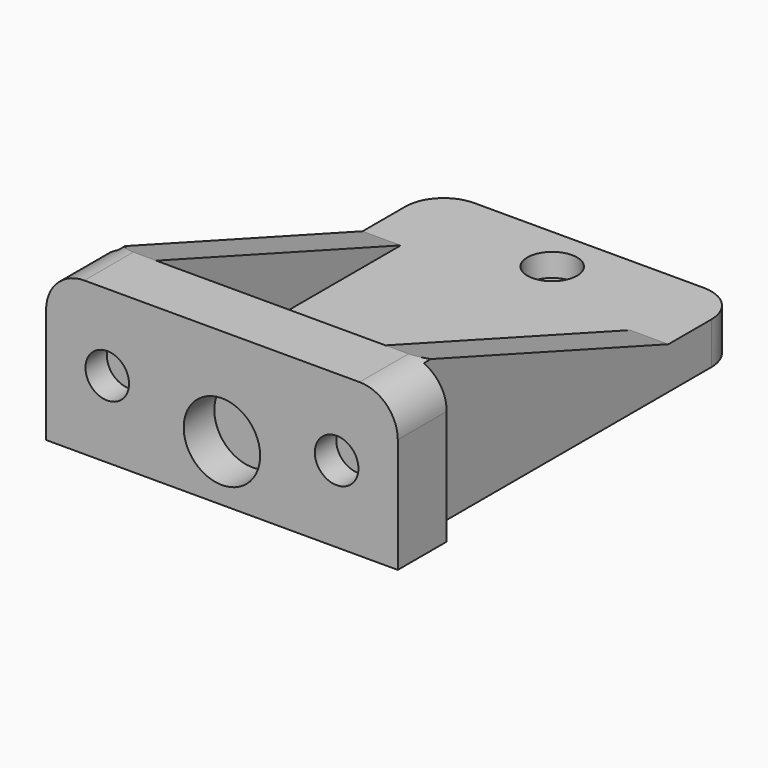
from build123d import *

# Parameters (mm, degrees)
F0_W           = 3
F0_H           = 8
F1_DEPTH       = 20
F0_W_2         = 30
F0_H_2         = 12
F0_H_3         = 40
F0_W_3         = 5
F2_DEPTH       = 5.5
F3_DEPTH       = 20
F5_DEPTH       = 43.001
F7_D           = 3.3
F7_DEPTH       = 13.5002857143
F7_CBORE_D     = 6.5
F7_CBORE_DEPTH = 3
F7_TIP         = 0.9914200214
F8_R           = 5
F9_DEPTH       = 5
F8_R_2         = 2.85
F10_DEPTH      = 3.5
F11_T1_DEPTH   = 30.5
F11_T3_DEPTH   = 33


# Not quite as in the source:
# - a fillet or chamfer that OpenCascade refuses, or shapes differently, is made with other operations: its cross-section is extruded or revolved along the edge and cut away or added


with BuildPart() as f1:
    # F0 (on Top) → F1 (new body)
    with BuildSketch(Plane.XY):
        Polygon((20, -30), (20, -22), (15, -22), (-15, -22), (-20, -22), (-20, -30), align=None)
        with Locations((-21.5, -26)):
            Rectangle(F0_W, F0_H)
        with Locations((21.5, -26)):
            Rectangle(F0_W, F0_H)
    extrude(amount=F1_DEPTH)

    # F0 (on Top) → F2 (join)
    with BuildSketch(Plane.XY):
        with Locations((0, 24)):
            Rectangle(F0_W_2, F0_H_2)
        with Locations((0, -2)):
            Rectangle(F0_W_2, F0_H_3)
        with Locations((-17.5, 24)):
            Rectangle(F0_W_3, F0_H_2)
        with Locations((-17.5, -2)):
            Rectangle(F0_W_3, F0_H_3)
        with Locations((17.5, 24)):
            Rectangle(F0_W_3, F0_H_2)
        with Locations((17.5, -2)):
            Rectangle(F0_W_3, F0_H_3)
    extrude(amount=F2_DEPTH)

    # F0 (on Top) → F3 (join)
    with BuildSketch(Plane.XY):
        with Locations((-17.5, -2)):
            Rectangle(F0_W_3, F0_H_3)
        with Locations((17.5, -2)):
            Rectangle(F0_W_3, F0_H_3)
    extrude(amount=F3_DEPTH)

    # F4 (on face) → F5 (cut, through all)
    with BuildSketch(Plane(origin=(-20, 0, 0), x_dir=(0, -1, 0), z_dir=(-1, 0, 0))):
        Polygon((-18, 20), (-18, 5.5), (22, 20), align=None)
    extrude(amount=-F5_DEPTH, mode=Mode.SUBTRACT)

    # F7
    with Locations(Plane.XY.offset(5.5)):
        with Locations((0, 24), (0, -16)):
            CounterBoreHole(F7_D / 2, F7_CBORE_D / 2, F7_CBORE_DEPTH, depth=F7_DEPTH)
            with Locations((0, 0, -(F7_DEPTH + F7_TIP / 2))):  # 118° drill point
                Cone(0, F7_D / 2, F7_TIP, mode=Mode.SUBTRACT)

    # F8 (on face) → F9 (cut)
    with BuildSketch(Plane.XZ.offset(30)):
        with Locations((0, 7.2906266057)):
            Circle(F8_R)
    extrude(amount=-F9_DEPTH, mode=Mode.SUBTRACT)

    # F8 (on face) → F10 (cut)
    with BuildSketch(Plane.XZ.offset(30)):
        with Locations((-15, 10)):
            Circle(F8_R_2)
        with Locations((15, 10)):
            Circle(F8_R_2)
    extrude(amount=-F10_DEPTH, mode=Mode.SUBTRACT)

    # F11: fillet of radius 5 on 4 edges, made by hand

    # F11_s2 → F11_t1 (cut)
    with BuildSketch(Plane.XY.offset(-12.5)):
        with BuildLine():
            ThreePointArc((15, 30), (18.5355339059, 28.5355339059), (20, 25))
            Line((20, 25), (20, 30))
            Line((20, 30), (15, 30))
        make_face()
        with BuildLine():
            ThreePointArc((-20, 25), (-18.5355339059, 28.5355339059), (-15, 30))
            Line((-15, 30), (-20, 30))
            Line((-20, 30), (-20, 25))
        make_face()
    extrude(amount=F11_T1_DEPTH, mode=Mode.SUBTRACT)

    # F11_s4 → F11_t3 (cut)
    with BuildSketch(Plane.XZ.offset(9.5)):
        with BuildLine():
            ThreePointArc((-23, 15), (-21.5355339059, 18.5355339059), (-18, 20))
            Line((-18, 20), (-23, 20))
            Line((-23, 20), (-23, 15))
        make_face()
        with BuildLine():
            ThreePointArc((18, 20), (21.5355339059, 18.5355339059), (23, 15))
            Line((23, 15), (23, 20))
            Line((23, 20), (18, 20))
        make_face()
    extrude(amount=F11_T3_DEPTH, mode=Mode.SUBTRACT)


solid = f1.part
